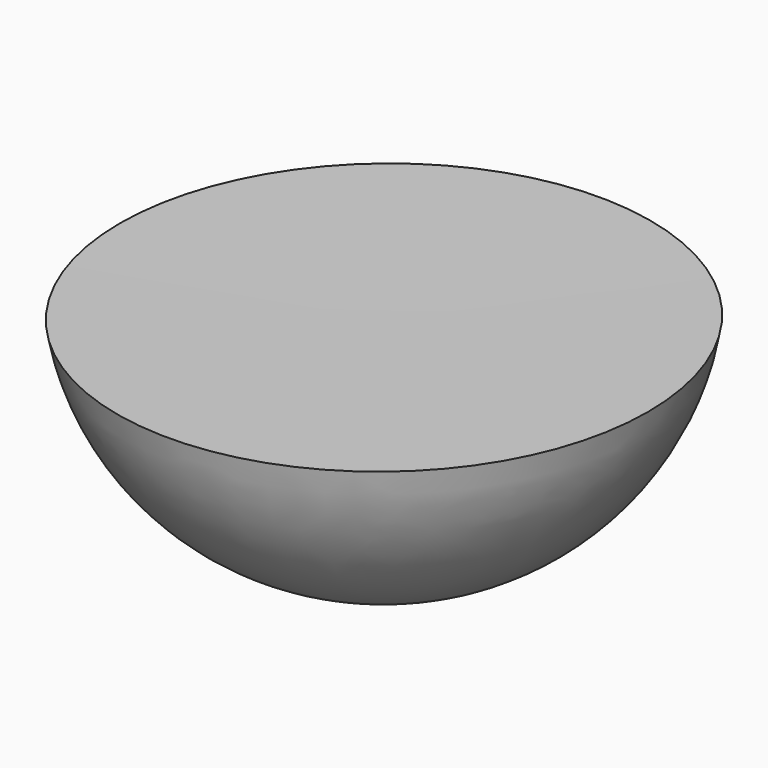
from build123d import *

# Parameters (mm, degrees)
F2_SCALE = 5


# Not quite as in the source:
# - a fillet or chamfer that OpenCascade refuses, or shapes differently, is made with other operations: its cross-section is extruded or revolved along the edge and cut away or added


with BuildPart() as f1:
    # F0 (on Front) → F1 (revolve)
    with BuildSketch(Plane.XZ):
        Polygon((45.9619096, 37.8984256), (-45.9619096, 36.2857288), (-45.1555612, -37.8984002), (45.9619096, -37.8984002), align=None)
    revolve(axis=Axis((-45.5587354, 0, -0.8063357), (-0.010868912, 0, 0.9999409316)))


with BuildPart() as f1_1:
    # F2: moved
    add(f1.part.scale(F2_SCALE))

    # F3: fillet of radius 449.015524587 on 2 edges, made by hand

    # F3_s1 → F3_t2 (revolve, cut)
    with BuildSketch(Plane.XZ):
        with BuildLine():
            ThreePointArc((229.809548, 189.492128), (77.982047099, -81.8414754589), (-213.7110771712, -189.492001))
            Line((-213.7110771712, -189.492001), (229.809548, -189.492001))
            Line((229.809548, -189.492001), (229.809548, 189.492128))
        make_face()
    revolve(axis=Axis((-225.723985986, 0, -194.4434473704), (-0.010868912, 0, 0.9999409316)), mode=Mode.SUBTRACT)


solid = f1_1.part
